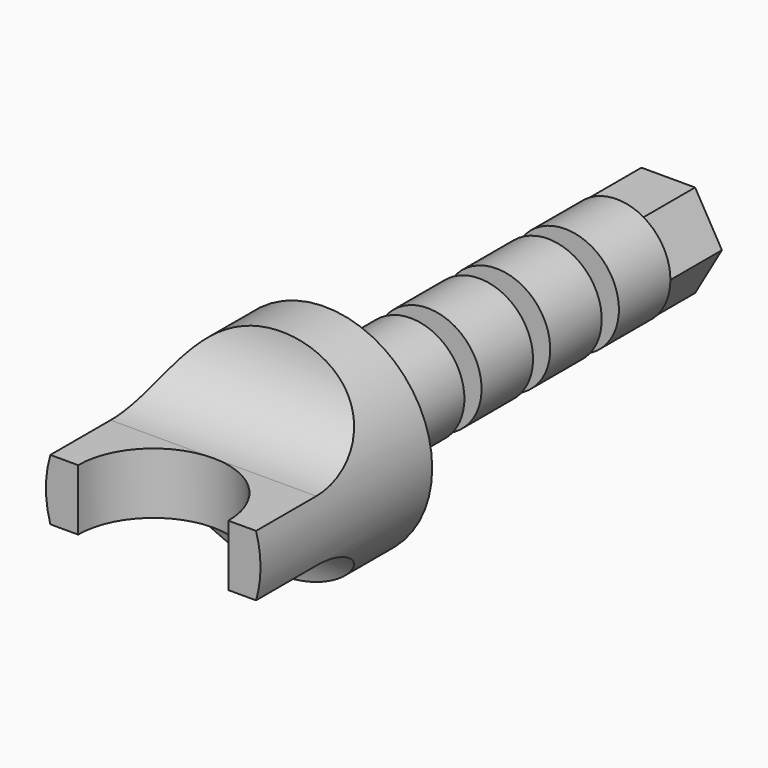
from build123d import *

# Parameters (mm, degrees)
F0_R          = 50
F1_DEPTH      = 100
F2_R          = 25
F3_DEPTH      = 50
F4_R          = 12.5
F5_DEPTH      = 10
F6_R          = 25
F7_DEPTH      = 30
F8_R          = 12.5
F9_DEPTH      = 10
F10_R         = 25
F11_DEPTH     = 30
F12_R         = 12.5
F13_DEPTH     = 10
F14_R         = 25
F15_DEPTH     = 30
F17_DEPTH     = 30
F20_D         = 70
F22_DEPTH     = 75
F23_T4_DEPTH  = 295.3549985752
F23_S5_R      = 50
F23_T6_DEPTH  = 152
F23_T10_DEPTH = 295.3549985752
F23_S11_R     = 50
F23_T12_DEPTH = 152


# Not quite as in the source:
# - a fillet or chamfer that OpenCascade refuses, or shapes differently, is made with other operations: its cross-section is extruded or revolved along the edge and cut away or added


with BuildPart() as f1:
    # F0 (on Front) → F1 (new body)
    with BuildSketch(Plane.XZ):
        Circle(F0_R)
    extrude(amount=F1_DEPTH)

    # F2 (on face) → F3 (join)
    with BuildSketch(Plane(origin=(0, 0, 0), x_dir=(-1, 0, 0), z_dir=(0, 1, 0))):
        Circle(F2_R)
    extrude(amount=F3_DEPTH)

    # F4 (on face) → F5 (join)
    with BuildSketch(Plane(origin=(0, 50, 0), x_dir=(-1, 0, 0), z_dir=(0, 1, 0))):
        Circle(F4_R)
    extrude(amount=F5_DEPTH)

    # F6 (on face) → F7 (join)
    with BuildSketch(Plane(origin=(0, 60, 0), x_dir=(-1, 0, 0), z_dir=(0, 1, 0))):
        Circle(F6_R)
    extrude(amount=F7_DEPTH)

    # F8 (on face) → F9 (join)
    with BuildSketch(Plane(origin=(0, 90, 0), x_dir=(-1, 0, 0), z_dir=(0, 1, 0))):
        Circle(F8_R)
    extrude(amount=F9_DEPTH)

    # F10 (on face) → F11 (join)
    with BuildSketch(Plane(origin=(0, 100, 0), x_dir=(-1, 0, 0), z_dir=(0, 1, 0))):
        Circle(F10_R)
    extrude(amount=F11_DEPTH)

    # F12 (on face) → F13 (join)
    with BuildSketch(Plane(origin=(0, 130, 0), x_dir=(-1, 0, 0), z_dir=(0, 1, 0))):
        Circle(F12_R)
    extrude(amount=F13_DEPTH)

    # F14 (on face) → F15 (join)
    with BuildSketch(Plane(origin=(0, 140, 0), x_dir=(-1, 0, 0), z_dir=(0, 1, 0))):
        Circle(F14_R)
    extrude(amount=F15_DEPTH)

    # F16 (on face) → F17 (join)
    with BuildSketch(Plane(origin=(0, 170, 0), x_dir=(-1, 0, 0), z_dir=(0, 1, 0))):
        Polygon((12.5, -21.6506350946), (25, 0), (12.5, 21.6506350946), (-12.5, 21.6506350946), (-25, 0), (-12.5, -21.6506350946), align=None)
    extrude(amount=F17_DEPTH)

    # F20 (through all)
    with Locations(Plane.XY.offset(50)):
        with Locations((0, -99.9434366822)):
            Hole(F20_D / 2)

    # F21 (on face) → F22 (cut)
    with BuildSketch(Plane.XZ.offset(100)):
        with BuildLine():
            ThreePointArc((47.9274992876, 14.2462209739), (0, 50), (-47.9274992876, 14.2462209739))
            Line((-47.9274992876, 14.2462209739), (47.9274992876, 14.2462209739))
        make_face()
        with BuildLine():
            Line((47.9274992876, -14.2462209739), (-47.9274992876, -14.2462209739))
            ThreePointArc((-47.9274992876, -14.2462209739), (0, -50), (47.9274992876, -14.2462209739))
        make_face()
    extrude(amount=-F22_DEPTH, mode=Mode.SUBTRACT)

    # F23: fillet of radius 39.9 on 2 edges, made by hand


with BuildPart() as f23_tool2:
    # F23_s3 → F23_t4 (new body)
    with BuildSketch(Plane.YZ.offset(-147.6774992876)):
        with BuildLine():
            ThreePointArc((-64.9, 14.2462209739), (-36.6864394307, 25.9326604046), (-25, 54.1462209739))
            Line((-25, 54.1462209739), (-25, 14.2462209739))
            Line((-25, 14.2462209739), (-64.9, 14.2462209739))
        make_face()
    extrude(amount=F23_T4_DEPTH)

    # F23_s5 → F23_t6 (intersect, symmetric)
    with BuildSketch(Plane.XZ.offset(44.9)):
        Circle(F23_S5_R)
    extrude(amount=F23_T6_DEPTH, both=True, mode=Mode.INTERSECT)


with BuildPart() as f1_1:
    add(f1.part)

    # F23_t1: union F23_tool2
    add(f23_tool2.part)


with BuildPart() as f23_tool8:
    # F23_s9 → F23_t10 (new body)
    with BuildSketch(Plane.YZ.offset(147.6774992876)):
        with BuildLine():
            ThreePointArc((-64.9, -14.2462209739), (-36.6864394307, -25.9326604046), (-25, -54.1462209739))
            Line((-25, -54.1462209739), (-25, -14.2462209739))
            Line((-25, -14.2462209739), (-64.9, -14.2462209739))
        make_face()
    extrude(amount=-F23_T10_DEPTH)

    # F23_s11 → F23_t12 (intersect, symmetric)
    with BuildSketch(Plane.XZ.offset(44.9)):
        Circle(F23_S11_R)
    extrude(amount=F23_T12_DEPTH, both=True, mode=Mode.INTERSECT)


with BuildPart() as f1_2:
    add(f1_1.part)

    # F23_t7: union F23_tool8
    add(f23_tool8.part)


solid = f1_2.part
